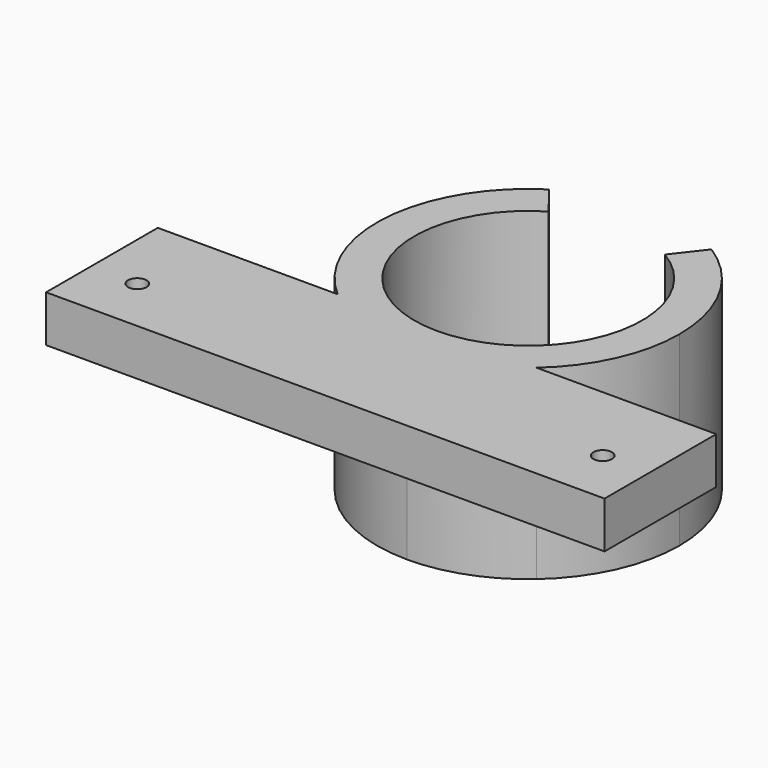
from build123d import *

# Parameters (mm, degrees)
F1_DEPTH = 40
F0_R     = 2
F2_DEPTH = 10


with BuildPart() as f1:
    # F0 (on Top) → F1 (new body)
    with BuildSketch(Plane.XY):
        with BuildLine():
            Line((-21.3541565041, -24.5), (0, -24.5))
            ThreePointArc((0, -24.5), (-23.6272833171, -6.4808551176), (-12.5, 21.0713075057))
            Line((-12.5, 21.0713075057), (-17.433109084, 27.4287569471))
            ThreePointArc((-17.433109084, 27.4287569471), (-32.4077451, 2.4470507823), (-21.3541565041, -24.5))
        make_face()
        with BuildLine():
            ThreePointArc((12.5, 21.0713075057), (21.289668856, 12.124355653), (24.5, 0))
            ThreePointArc((24.5, 0), (17.3241161391, -17.3241161391), (0, -24.5))
            Line((0, -24.5), (21.3541565041, -24.5))
            ThreePointArc((21.3541565041, -24.5), (29.582596965, -13.4580814684), (32.5, 0))
            ThreePointArc((32.5, 0), (28.4853124016, 15.6472674095), (17.433109084, 27.4287569471))
            Line((17.433109084, 27.4287569471), (12.5, 21.0713075057))
        make_face()
        with BuildLine():
            Line((21.3541565041, -24.5), (0, -24.5))
            Line((0, -24.5), (0, -32.5))
            ThreePointArc((0, -32.5), (11.401754251, -30.4343555871), (21.3541565041, -24.5))
        make_face()
        with BuildLine():
            Line((0, -32.5), (0, -24.5))
            Line((0, -24.5), (-21.3541565041, -24.5))
            ThreePointArc((-21.3541565041, -24.5), (-11.401754251, -30.4343555871), (0, -32.5))
        make_face()
    extrude(amount=-F1_DEPTH)

    # F0 (on Top) → F2 (join)
    with BuildSketch(Plane.XY):
        with BuildLine():
            Line((0, -54.5), (0, -32.5))
            ThreePointArc((0, -32.5), (-11.401754251, -30.4343555871), (-21.3541565041, -24.5))
            Line((-21.3541565041, -24.5), (-60, -24.5))
            Line((-60, -24.5), (-60, -54.5))
            Line((-60, -54.5), (0, -54.5))
        make_face()
        with Locations((-50.0000007451, -42.5000099838)):
            Circle(F0_R, mode=Mode.SUBTRACT)
        with BuildLine():
            ThreePointArc((21.3541565041, -24.5), (11.401754251, -30.4343555871), (0, -32.5))
            Line((0, -32.5), (0, -54.5))
            Line((0, -54.5), (60, -54.5))
            Line((60, -54.5), (60, -24.5))
            Line((60, -24.5), (21.3541565041, -24.5))
        make_face()
        with Locations((50.0000007451, -42.5000099838)):
            Circle(F0_R, mode=Mode.SUBTRACT)
    extrude(amount=-F2_DEPTH)


solid = f1.part
